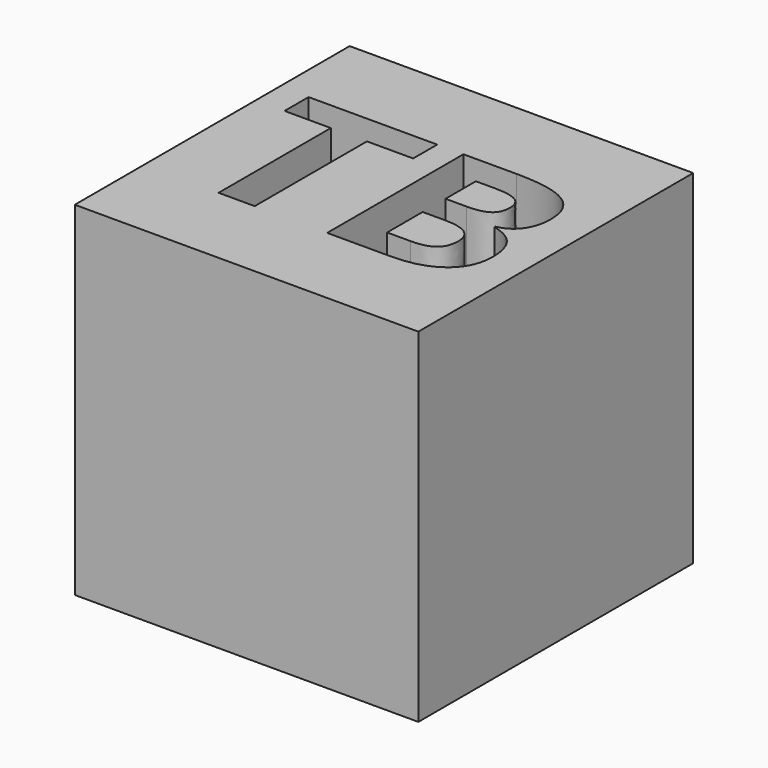
from build123d import *

# Parameters (mm, degrees)
F0_W         = 25.4
F0_H         = 25.4
F1_DEPTH     = 25.4
F2_TEXT_SIZE = 17.6388888889
F3_DEPTH     = 6.35
F4_TEXT_SIZE = 15.1218604651
F5_DEPTH     = 6.35


# Not quite as in the source:
# - Text() gives the source's letters only with a copy of the font that has no kerning and outlines rounded to 1/6400 em; it was checked with that copy


with BuildPart() as f1:
    # F0 (on Top) → F1 (new body)
    with BuildSketch(Plane.XY):
        with Locations((12.7, 12.7)):
            Rectangle(F0_W, F0_H)
    extrude(amount=F1_DEPTH)

    # F2 (on face) → F3 (cut)
    with BuildSketch(Plane.XY.offset(25.4)):
        with Locations((1.778, 6.35)):
            Text('TB', F2_TEXT_SIZE, font='Open Sans', font_style=FontStyle.BOLD, text_align=(TextAlign.LEFT, TextAlign.BOTTOM))
    extrude(amount=-F3_DEPTH, mode=Mode.SUBTRACT)

    # F4 (on face) → F5 (cut)
    with BuildSketch(Plane(origin=(0, 0, 0), x_dir=(1, 0, 0), z_dir=(0, 0, -1))):
        with Locations((1.524, -17.2377395349)):
            Text('DQ', F4_TEXT_SIZE, font='Open Sans', text_align=(TextAlign.LEFT, TextAlign.BOTTOM))
    extrude(amount=-F5_DEPTH, mode=Mode.SUBTRACT)


solid = f1.part
